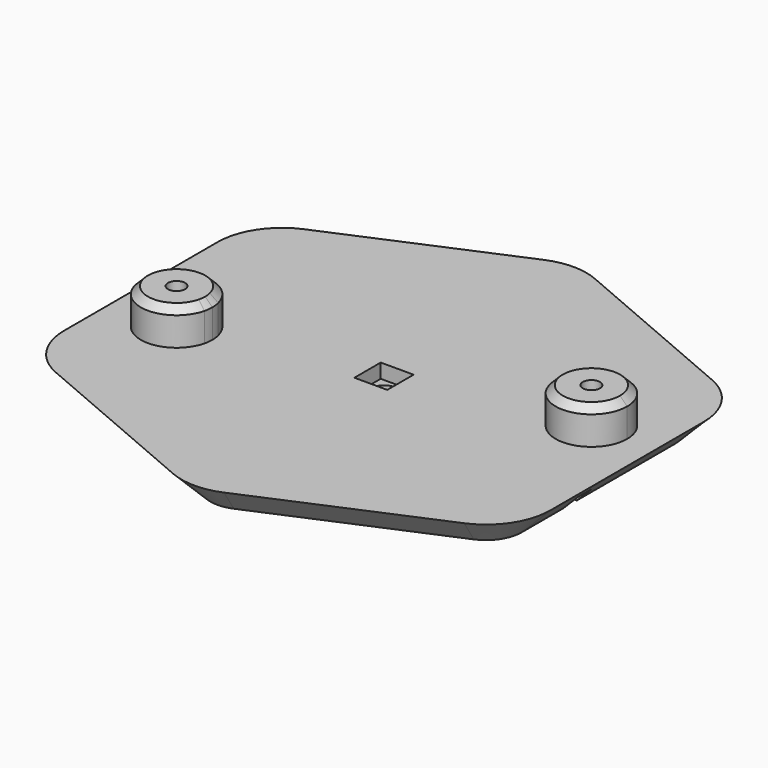
from build123d import *

# Parameters (mm, degrees)
F0_W           = 25
F0_H           = 6.3
F0_H_2         = 2.4
F0_H_3         = 7.6
F0_R           = 1.7
F0_W_2         = 22.5
F1_DEPTH       = 4
F2_DEPTH       = 9
F3_DEPTH       = 2.1
F4_DEPTH       = 4
F5_T1_DEPTH    = 50.7168298797
F5_T3_DEPTH    = 50.7168298797
F5_2_T1_DEPTH  = 27.1991896638
F5_2_T3_DEPTH  = 20.06445336
F5_2_T5_DEPTH  = 27.1991896638
F5_2_T7_DEPTH  = 30.06445336
F5_2_T9_DEPTH  = 27.1991896638
F5_2_T11_DEPTH = 20.06445336
F5_2_T13_DEPTH = 27.1991896638
F5_2_T15_DEPTH = 30.06445336
F5_2_T18_ANGLE = 66.8014094864
F5_2_T20_ANGLE = 46.3971810273
F5_2_T22_ANGLE = 66.8014094864
F5_2_T24_ANGLE = 66.8014094864
F5_2_T26_ANGLE = 46.3971810273
F5_2_T28_ANGLE = 66.8014094864
F6_SIZE        = 1
F7_W           = 4.6
F7_H           = 4.6
F7_R           = 1.7
F8_DEPTH       = 2


# Not quite as in the source:
# - a fillet or chamfer that OpenCascade refuses, or shapes differently, is made with other operations: its cross-section is extruded or revolved along the edge and cut away or added


with BuildPart() as f1:
    # F0 (on Top) → F1 (new body)
    with BuildSketch(Plane.XY):
        with BuildLine():
            Line((-12.5, -3.8), (-12.5, 3.8))
            Line((-12.5, 3.8), (-35, 3.8))
            Line((-35, 3.8), (-35, 0.3032439272))
            Line((-35, 0.3032439272), (-35, -0.3032439272))
            Line((-35, -0.3032439272), (-35, -13.4060384202))
            ThreePointArc((-35, -13.4060384202), (-33.3484109224, -18.9109485077), (-28.9391929858, -22.5974887204))
            Line((-28.9391929858, -22.5974887204), (-3.9391929858, -33.3117744347))
            ThreePointArc((-3.9391929858, -33.3117744347), (0, -34.1203241345), (3.9391929858, -33.3117744347))
            Line((3.9391929858, -33.3117744347), (28.9391929858, -22.5974887204))
            ThreePointArc((28.9391929858, -22.5974887204), (33.3484109224, -18.9109485077), (35, -13.4060384202))
            Line((35, -13.4060384202), (35, -6.2))
            Line((35, -6.2), (12.5, -6.2))
            Line((12.5, -6.2), (12.5, -12.5))
            Line((12.5, -12.5), (-12.5, -12.5))
            Line((-12.5, -12.5), (-12.5, -6.2))
            Line((-12.5, -6.2), (-20.1461355602, -6.2))
            ThreePointArc((-20.1461355602, -6.2), (-30, -5), (-20.1461355602, -3.8))
            Line((-20.1461355602, -3.8), (-12.5, -3.8))
        make_face()
        with BuildLine():
            ThreePointArc((20.1461355602, 6.2), (25.6044327096, 9.9633316532), (30, 5))
            ThreePointArc((30, 5), (25.6044327096, 0.0366683468), (20.1461355602, 3.8))
            Line((20.1461355602, 3.8), (12.5, 3.8))
            Line((12.5, 3.8), (12.5, -3.8))
            Line((12.5, -3.8), (35, -3.8))
            Line((35, -3.8), (35, -0.49606018))
            Line((35, -0.49606018), (35, 0.49606018))
            Line((35, 0.49606018), (35, 13.4060384202))
            ThreePointArc((35, 13.4060384202), (33.3484109224, 18.9109485077), (28.9391929858, 22.5974887204))
            Line((28.9391929858, 22.5974887204), (3.9391929858, 33.3117744347))
            ThreePointArc((3.9391929858, 33.3117744347), (0, 34.1203241345), (-3.9391929858, 33.3117744347))
            Line((-3.9391929858, 33.3117744347), (-28.9391929858, 22.5974887204))
            ThreePointArc((-28.9391929858, 22.5974887204), (-33.3484109224, 18.9109485077), (-35, 13.4060384202))
            Line((-35, 13.4060384202), (-35, 6.2))
            Line((-35, 6.2), (-12.5, 6.2))
            Line((-12.5, 6.2), (-12.5, 12.5))
            Line((-12.5, 12.5), (12.5, 12.5))
            Line((12.5, 12.5), (12.5, 6.2))
            Line((12.5, 6.2), (20.1461355602, 6.2))
        make_face()
        with BuildLine():
            ThreePointArc((20.1461355602, 3.8), (25.6044327096, 0.0366683468), (30, 5))
            ThreePointArc((30, 5), (25.6044327096, 9.9633316532), (20.1461355602, 6.2))
            Line((20.1461355602, 6.2), (25, 6.2))
            ThreePointArc((25, 6.2), (25.8485281374, 5.8485281374), (26.2, 5))
            ThreePointArc((26.2, 5), (25.8485281374, 4.1514718626), (25, 3.8))
            Line((25, 3.8), (20.1461355602, 3.8))
        make_face()
        with BuildLine():
            Line((25, 6.2), (20.1461355602, 6.2))
            ThreePointArc((20.1461355602, 6.2), (20, 5), (20.1461355602, 3.8))
            Line((20.1461355602, 3.8), (25, 3.8))
            ThreePointArc((25, 3.8), (23.8, 5), (25, 6.2))
        make_face()
        with BuildLine():
            ThreePointArc((20.1461355602, 3.8), (20, 5), (20.1461355602, 6.2))
            Line((20.1461355602, 6.2), (12.5, 6.2))
            Line((12.5, 6.2), (12.5, 3.8))
            Line((12.5, 3.8), (20.1461355602, 3.8))
        make_face()
        with Locations((0, 9.35)):
            Rectangle(F0_W, F0_H)
        with Locations((0, 5)):
            Rectangle(F0_W, F0_H_2)
        Rectangle(F0_W, F0_H_3)
        Circle(F0_R, mode=Mode.SUBTRACT)
        with Locations((-23.75, 5)):
            Rectangle(F0_W_2, F0_H_2)
        with BuildLine():
            Line((-25, -3.8), (-20.1461355602, -3.8))
            ThreePointArc((-20.1461355602, -3.8), (-30, -5), (-20.1461355602, -6.2))
            Line((-20.1461355602, -6.2), (-25, -6.2))
            ThreePointArc((-25, -6.2), (-26.2, -5), (-25, -3.8))
        make_face()
        with BuildLine():
            ThreePointArc((-20, -5), (-20.0366683468, -4.3955672904), (-20.1461355602, -3.8))
            Line((-20.1461355602, -3.8), (-25, -3.8))
            ThreePointArc((-25, -3.8), (-24.1514718626, -4.1514718626), (-23.8, -5))
            ThreePointArc((-23.8, -5), (-24.1514718626, -5.8485281374), (-25, -6.2))
            Line((-25, -6.2), (-20.1461355602, -6.2))
            ThreePointArc((-20.1461355602, -6.2), (-20.0366683468, -5.6044327096), (-20, -5))
        make_face()
        with Locations((23.75, -5)):
            Rectangle(F0_W_2, F0_H_2)
        with Locations((0, -9.35)):
            Rectangle(F0_W, F0_H)
        with BuildLine():
            Line((-12.5, -6.2), (-12.5, -3.8))
            Line((-12.5, -3.8), (-20.1461355602, -3.8))
            ThreePointArc((-20.1461355602, -3.8), (-20.0366683468, -4.3955672904), (-20, -5))
            ThreePointArc((-20, -5), (-20.0366683468, -5.6044327096), (-20.1461355602, -6.2))
            Line((-20.1461355602, -6.2), (-12.5, -6.2))
        make_face()
        with Locations((0, -5)):
            Rectangle(F0_W, F0_H_2)
    extrude(amount=F1_DEPTH)

    # F0 (on Top) → F2 (join)
    with BuildSketch(Plane.XY):
        with BuildLine():
            Line((-25, -3.8), (-20.1461355602, -3.8))
            ThreePointArc((-20.1461355602, -3.8), (-30, -5), (-20.1461355602, -6.2))
            Line((-20.1461355602, -6.2), (-25, -6.2))
            ThreePointArc((-25, -6.2), (-26.2, -5), (-25, -3.8))
        make_face()
        with BuildLine():
            ThreePointArc((20.1461355602, 3.8), (25.6044327096, 0.0366683468), (30, 5))
            ThreePointArc((30, 5), (25.6044327096, 9.9633316532), (20.1461355602, 6.2))
            Line((20.1461355602, 6.2), (25, 6.2))
            ThreePointArc((25, 6.2), (25.8485281374, 5.8485281374), (26.2, 5))
            ThreePointArc((26.2, 5), (25.8485281374, 4.1514718626), (25, 3.8))
            Line((25, 3.8), (20.1461355602, 3.8))
        make_face()
        with BuildLine():
            Line((25, 6.2), (20.1461355602, 6.2))
            ThreePointArc((20.1461355602, 6.2), (20, 5), (20.1461355602, 3.8))
            Line((20.1461355602, 3.8), (25, 3.8))
            ThreePointArc((25, 3.8), (23.8, 5), (25, 6.2))
        make_face()
        with BuildLine():
            ThreePointArc((-20, -5), (-20.0366683468, -4.3955672904), (-20.1461355602, -3.8))
            Line((-20.1461355602, -3.8), (-25, -3.8))
            ThreePointArc((-25, -3.8), (-24.1514718626, -4.1514718626), (-23.8, -5))
            ThreePointArc((-23.8, -5), (-24.1514718626, -5.8485281374), (-25, -6.2))
            Line((-25, -6.2), (-20.1461355602, -6.2))
            ThreePointArc((-20.1461355602, -6.2), (-20.0366683468, -5.6044327096), (-20, -5))
        make_face()
    extrude(amount=F2_DEPTH)

    # F0 (on Top) → F3 (cut)
    with BuildSketch(Plane.XY):
        with BuildLine():
            ThreePointArc((-20, -5), (-20.0366683468, -4.3955672904), (-20.1461355602, -3.8))
            Line((-20.1461355602, -3.8), (-25, -3.8))
            ThreePointArc((-25, -3.8), (-24.1514718626, -4.1514718626), (-23.8, -5))
            ThreePointArc((-23.8, -5), (-24.1514718626, -5.8485281374), (-25, -6.2))
            Line((-25, -6.2), (-20.1461355602, -6.2))
            ThreePointArc((-20.1461355602, -6.2), (-20.0366683468, -5.6044327096), (-20, -5))
        make_face()
        with BuildLine():
            Line((-12.5, -6.2), (-12.5, -3.8))
            Line((-12.5, -3.8), (-20.1461355602, -3.8))
            ThreePointArc((-20.1461355602, -3.8), (-20.0366683468, -4.3955672904), (-20, -5))
            ThreePointArc((-20, -5), (-20.0366683468, -5.6044327096), (-20.1461355602, -6.2))
            Line((-20.1461355602, -6.2), (-12.5, -6.2))
        make_face()
        with Locations((0, -5)):
            Rectangle(F0_W, F0_H_2)
        with Locations((23.75, -5)):
            Rectangle(F0_W_2, F0_H_2)
        with BuildLine():
            Line((25, 6.2), (20.1461355602, 6.2))
            ThreePointArc((20.1461355602, 6.2), (20, 5), (20.1461355602, 3.8))
            Line((20.1461355602, 3.8), (25, 3.8))
            ThreePointArc((25, 3.8), (23.8, 5), (25, 6.2))
        make_face()
        with BuildLine():
            ThreePointArc((20.1461355602, 3.8), (20, 5), (20.1461355602, 6.2))
            Line((20.1461355602, 6.2), (12.5, 6.2))
            Line((12.5, 6.2), (12.5, 3.8))
            Line((12.5, 3.8), (20.1461355602, 3.8))
        make_face()
        with Locations((0, 5)):
            Rectangle(F0_W, F0_H_2)
        with Locations((-23.75, 5)):
            Rectangle(F0_W_2, F0_H_2)
    extrude(amount=F3_DEPTH, mode=Mode.SUBTRACT)

    # F5#2: chamfer of 5 on 2 edges, made by hand

    # F5_2_s2 → F5_2_t1 (cut)
    with BuildSketch(Plane(origin=(8.7332208073, 3.7428089174, 0), x_dir=(0, 0, 1), z_dir=(-0.91914503, -0.3939192986, 0))):
        Polygon((0, 27.1700760506), (5, 32.1700760506), (0, 32.1700760506), align=None)
    extrude(amount=F5_2_T1_DEPTH, mode=Mode.SUBTRACT)

    # F5_2_s4 → F5_2_t3 (cut)
    with BuildSketch(Plane.XZ.offset(-13.4060384202)):
        Polygon((-30, 0), (-35, 5), (-35, 0), align=None)
    extrude(amount=F5_2_T3_DEPTH, mode=Mode.SUBTRACT)

    # F5_2_s6 → F5_2_t5 (cut)
    with BuildSketch(Plane(origin=(16.2667791927, -6.9714767969, 0), x_dir=(0, 0, 1), z_dir=(-0.91914503, 0.3939192986, 0))):
        Polygon((5, 32.1700760506), (0, 27.1700760506), (0, 32.1700760506), align=None)
    extrude(amount=F5_2_T5_DEPTH, mode=Mode.SUBTRACT)

    # F5_2_s8 → F5_2_t7 (cut)
    with BuildSketch(Plane.XZ.offset(-13.4060384202)):
        Polygon((35, 5), (30, 0), (35, 0), align=None)
    extrude(amount=F5_2_T7_DEPTH, mode=Mode.SUBTRACT)

    # F5_2_s10 → F5_2_t9 (cut)
    with BuildSketch(Plane(origin=(-8.7332208073, -3.7428089174, 0), x_dir=(0, 0, 1), z_dir=(0.91914503, 0.3939192986, 0))):
        Polygon((0, 27.1700760506), (5, 32.1700760506), (0, 32.1700760506), align=None)
    extrude(amount=F5_2_T9_DEPTH, mode=Mode.SUBTRACT)

    # F5_2_s12 → F5_2_t11 (cut)
    with BuildSketch(Plane.XZ.offset(-6.6584149398)):
        Polygon((35, 5), (30, 0), (35, 0), align=None)
    extrude(amount=F5_2_T11_DEPTH, mode=Mode.SUBTRACT)

    # F5_2_s14 → F5_2_t13 (cut)
    with BuildSketch(Plane(origin=(-16.2667791927, 6.9714767969, 0), x_dir=(0, 0, 1), z_dir=(0.91914503, -0.3939192986, 0))):
        Polygon((0, 27.1700760506), (5, 32.1700760506), (0, 32.1700760506), align=None)
    extrude(amount=F5_2_T13_DEPTH, mode=Mode.SUBTRACT)

    # F5_2_s16 → F5_2_t15 (cut)
    with BuildSketch(Plane.XZ.offset(-16.6584149398)):
        Polygon((-30, 0), (-35, 5), (-35, 0), align=None)
    extrude(amount=F5_2_T15_DEPTH, mode=Mode.SUBTRACT)

    # F5_2_s17 → F5_2_t18 (revolve, cut)
    with BuildSketch(Plane(origin=(16.2667791927, 6.9714767969, 0), x_dir=(0, 0, 1), z_dir=(-0.91914503, -0.3939192986, 0))):
        Polygon((0, -27.1700760506), (5, -32.1700760506), (0, -32.1700760506), align=None)
    revolve(axis=Axis((25, -13.4060384202, 0), (0, 0, 1)), revolution_arc=F5_2_T18_ANGLE, mode=Mode.SUBTRACT)

    # F5_2_s19 → F5_2_t20 (revolve, cut)
    with BuildSketch(Plane(origin=(-8.7332208073, 3.7428089174, 0), x_dir=(0, 0, 1), z_dir=(0.91914503, -0.3939192986, 0))):
        Polygon((0, -27.1700760506), (5, -32.1700760506), (0, -32.1700760506), align=None)
    revolve(axis=Axis((0, 24.1203241345, 0), (0, 0, 1)), revolution_arc=F5_2_T20_ANGLE, mode=Mode.SUBTRACT)

    # F5_2_s21 → F5_2_t22 (revolve, cut)
    with BuildSketch(Plane(origin=(-16.2667791927, -6.9714767969, 0), x_dir=(0, 0, 1), z_dir=(0.91914503, 0.3939192986, 0))):
        Polygon((0, -27.1700760506), (5, -32.1700760506), (0, -32.1700760506), align=None)
    revolve(axis=Axis((-25, 13.4060384202, 0), (0, 0, 1)), revolution_arc=F5_2_T22_ANGLE, mode=Mode.SUBTRACT)

    # F5_2_s23 → F5_2_t24 (revolve, cut)
    with BuildSketch(Plane.XZ.offset(-13.4060384202)):
        Polygon((35, 5), (30, 0), (35, 0), align=None)
    revolve(axis=Axis((25, 13.4060384202, 0), (0, 0, 1)), revolution_arc=F5_2_T24_ANGLE, mode=Mode.SUBTRACT)

    # F5_2_s25 → F5_2_t26 (revolve, cut)
    with BuildSketch(Plane(origin=(8.7332208073, -3.7428089174, 0), x_dir=(0, 0, 1), z_dir=(-0.91914503, 0.3939192986, 0))):
        Polygon((0, -27.1700760506), (5, -32.1700760506), (0, -32.1700760506), align=None)
    revolve(axis=Axis((0, -24.1203241345, 0), (0, 0, 1)), revolution_arc=F5_2_T26_ANGLE, mode=Mode.SUBTRACT)

    # F5_2_s27 → F5_2_t28 (revolve, cut)
    with BuildSketch(Plane.XZ.offset(13.4060384202)):
        Polygon((-30, 0), (-35, 5), (-35, 0), align=None)
    revolve(axis=Axis((-25, -13.4060384202, 0), (0, 0, 1)), revolution_arc=F5_2_T28_ANGLE, mode=Mode.SUBTRACT)

    # F6
    f6_edges = [f1.edges().sort_by_distance(p)[0] for p in [
        (29.853864, 3.8, 9),
        (-29.853864, -3.8, 9),
    ]]
    chamfer(f6_edges, length=F6_SIZE)

    # F7 (on face) → F8 (cut)
    with BuildSketch(Plane.XY.offset(4)):
        Rectangle(F7_W, F7_H)
        Circle(F7_R, mode=Mode.SUBTRACT)
    extrude(amount=-F8_DEPTH, mode=Mode.SUBTRACT)


with BuildPart() as f4:
    # F0 (on Top) → F4 (new body)
    with BuildSketch(Plane.XY):
        with Locations((0, -9.35)):
            Rectangle(F0_W, F0_H)
        with Locations((0, -5)):
            Rectangle(F0_W, F0_H_2)
        Rectangle(F0_W, F0_H_3)
        Circle(F0_R, mode=Mode.SUBTRACT)
        with Locations((0, 5)):
            Rectangle(F0_W, F0_H_2)
        with Locations((0, 9.35)):
            Rectangle(F0_W, F0_H)
    extrude(amount=-F4_DEPTH)

    # F5: chamfer of 5 on 4 edges, made by hand

    # F5_s2 → F5_t1 (cut)
    with BuildSketch(Plane.XZ.offset(-25.3584149398)):
        Polygon((12.5, 1), (7.5, -4), (12.5, -4), align=None)
        Polygon((-12.5, 1), (-7.5, -4), (-12.5, -4), align=None)
    extrude(amount=F5_T1_DEPTH, mode=Mode.SUBTRACT)

    # F5_s4 → F5_t3 (cut)
    with BuildSketch(Plane.YZ.offset(-25.3584149398)):
        Polygon((-12.5, 1), (-7.5, -4), (-12.5, -4), align=None)
        Polygon((12.5, 1), (7.5, -4), (12.5, -4), align=None)
    extrude(amount=F5_T3_DEPTH, mode=Mode.SUBTRACT)


solid = Compound([f1.part, f4.part])
